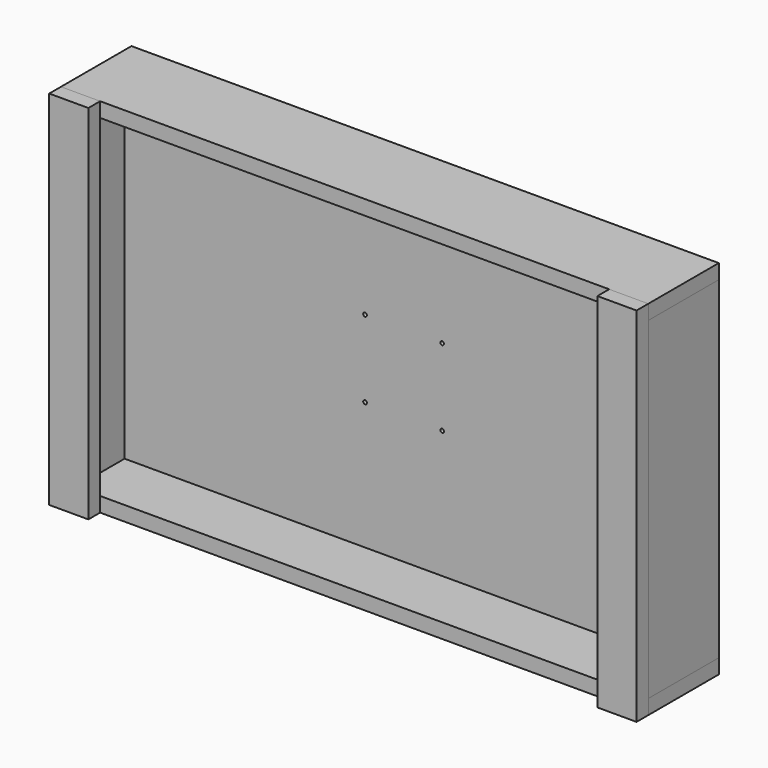
from build123d import *

# Parameters (mm, degrees)
F4_DEPTH       = 114.3
F5_W           = 6.35
F5_H           = 9.525
F6_DEPTH       = 234.951
F6_DEPTH_BACK  = 234.951
F8_DEPTH       = 19.05
F10_DEPTH      = 25.4
F12_DEPTH      = 723.9
F13_R          = 2.38125
F14_DEPTH      = 12.7
F15_W          = 736.6
F15_H          = 9.525
F16_DEPTH      = 215.9
F16_DEPTH_BACK = 215.9
F18_R          = 2.38125
F19_DEPTH      = 34.926


with BuildPart() as f4:
    # F1 (on Front) → F4 (new body)
    with BuildSketch(Plane.XZ):
        Polygon((381, 234.95), (-381, 234.95), (-381, 215.9), (-371.475, 215.9), (-371.475, 225.425), (-361.95, 225.425), (-361.95, 215.9), (361.95, 215.9), (361.95, 225.425), (371.475, 225.425), (371.475, 215.9), (381, 215.9), align=None)
    extrude(amount=F4_DEPTH)


with BuildPart() as f4b:
    # F3 (on Front) → F4, piece 2 (new body)
    with BuildSketch(Plane.XZ):
        Polygon((-371.475, 215.9), (-381, 215.9), (-381, -215.9), (-371.475, -215.9), (-371.475, -225.425), (-361.95, -225.425), (-361.95, -215.9), (-361.95, 215.9), (-361.95, 225.425), (-371.475, 225.425), align=None)
    extrude(amount=F4_DEPTH)


with BuildPart() as f4c:
    # F3 (on Front) → F4, piece 3 (new body)
    with BuildSketch(Plane.XZ):
        Polygon((381, 215.9), (371.475, 215.9), (371.475, 225.425), (361.95, 225.425), (361.95, 215.9), (361.95, -215.9), (361.95, -225.425), (371.475, -225.425), (371.475, -215.9), (381, -215.9), align=None)
    extrude(amount=F4_DEPTH)


with BuildPart() as f4d:
    # F2 (on Front) → F4, piece 4 (new body)
    with BuildSketch(Plane.XZ):
        Polygon((-381, -215.9), (-381, -234.95), (381, -234.95), (381, -215.9), (371.475, -215.9), (371.475, -225.425), (361.95, -225.425), (361.95, -215.9), (-361.95, -215.9), (-361.95, -225.425), (-371.475, -225.425), (-371.475, -215.9), align=None)
    extrude(amount=F4_DEPTH)

    # F9 (on face) → F10 (cut)
    with BuildSketch(Plane.XY.offset(-215.9)):
        with BuildLine():
            Line((50.8, 0), (-50.8, 0))
            Line((-50.8, 0), (-50.8, -12.7))
            ThreePointArc((-50.8, -12.7), (-47.0802561211, -21.6802561211), (-38.1, -25.4))
            Line((-38.1, -25.4), (38.1, -25.4))
            ThreePointArc((38.1, -25.4), (47.0802561211, -21.6802561211), (50.8, -12.7))
            Line((50.8, -12.7), (50.8, 0))
        make_face()
    extrude(amount=-F10_DEPTH, mode=Mode.SUBTRACT)


with BuildPart() as f6_tool:
    # F5 (on Top) → F6 (new body, two sides)
    with BuildSketch(Plane.XY) as f6_sk:
        with Locations((-365.125, -30.1625)):
            Rectangle(F5_W, F5_H)
        with Locations((365.125, -30.1625)):
            Rectangle(F5_W, F5_H)
    extrude(amount=-F6_DEPTH)
    extrude(f6_sk.sketch, amount=F6_DEPTH_BACK)


with BuildPart() as f4b_1:
    add(f4b.part)

    # F6: cut by f6_tool
    add(f6_tool.part, mode=Mode.SUBTRACT)


with BuildPart() as f4c_1:
    add(f4c.part)

    # F6: cut by f6_tool
    add(f6_tool.part, mode=Mode.SUBTRACT)


with BuildPart() as f8:
    # F7 (on face) → F8 (new body)
    with BuildSketch(Plane.XZ.offset(114.3)):
        Polygon((361.95, 215.9), (330.2, 215.9), (330.2, -234.95), (381, -234.95), (381, 215.9), (371.475, 215.9), (371.475, 225.425), (361.95, 225.425), align=None)
        Polygon((381, 234.95), (330.2, 234.95), (330.2, 215.9), (361.95, 215.9), (361.95, 225.425), (371.475, 225.425), (371.475, 215.9), (381, 215.9), align=None)
    extrude(amount=F8_DEPTH)

    # F13 (on face) → F14 (cut)
    with BuildSketch(Plane(origin=(0, -114.3, 0), x_dir=(-1, 0, 0), z_dir=(0, 1, 0))):
        with Locations((-338.9122, 162.71875)):
            Circle(F13_R)
        with Locations((-338.9122, -162.71875)):
            Circle(F13_R)
    extrude(amount=-F14_DEPTH, mode=Mode.SUBTRACT)


with BuildPart() as f12:
    # F11 (on face) → F12 (new body, through all)
    with BuildSketch(Plane(origin=(361.95, 0, 0), x_dir=(0, -1, 0), z_dir=(-1, 0, 0))):
        Polygon((19.05, 215.9), (0, 215.9), (0, 165.1), (19.05, 184.15), align=None)
    extrude(amount=F12_DEPTH)


with BuildPart() as f16:
    # F15 (on Top) → F16 (new body, two sides)
    with BuildSketch(Plane.XY) as f16_sk:
        with Locations((0, -30.1625)):
            Rectangle(F15_W, F15_H)
    extrude(amount=F16_DEPTH)
    extrude(f16_sk.sketch, amount=-F16_DEPTH_BACK)

    # F18 (on face) → F19 (cut, through all)
    with BuildSketch(Plane.XZ.offset(34.925)):
        with Locations((-50, 50)):
            Circle(F18_R)
        with Locations((50, 50)):
            Circle(F18_R)
        with Locations((-50, -50)):
            Circle(F18_R)
        with Locations((50, -50)):
            Circle(F18_R)
    extrude(amount=-F19_DEPTH, mode=Mode.SUBTRACT)


with BuildPart() as f17_1:
    # F17: instance of F8
    add(f8.part.mirror(Plane.YZ))


solid = Compound([f4.part, f4d.part, f4b_1.part, f4c_1.part, f8.part, f12.part, f16.part, f17_1.part])
